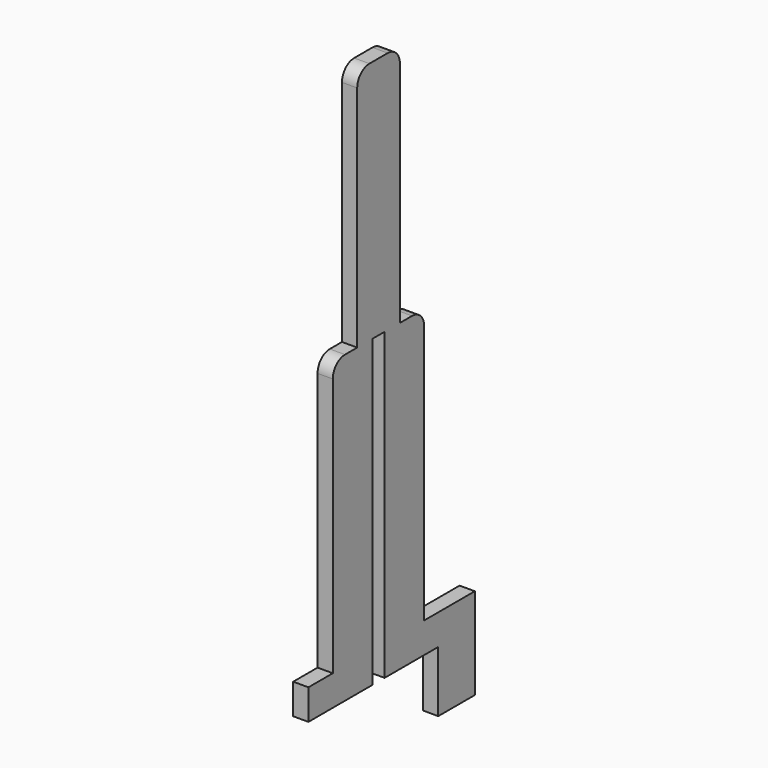
from build123d import *

# Parameters (mm, degrees)
F1_DEPTH = 3.175


# Not quite as in the source:
# - ends of sketch curves that miss each other by under 0.0002 mm in the source are joined


with BuildPart() as f1:
    # F0 (on Right) → F1 (new body, symmetric)
    with BuildSketch(Plane.YZ):
        with BuildLine():
            Line((3.175, -63.5), (23.8125, -63.5))
            Line((23.8125, -63.5), (23.8125, -50.8))
            Line((23.8125, -50.8), (23.8125, 57.15))
            ThreePointArc((23.8125, 57.15), (21.9533763667, 61.6393796296), (17.4646167058, 63.4999996472))
            Line((17.4646167058, 63.4999996472), (17.4625, 63.5))
            Line((17.4625, 63.5), (11.1139111112, 63.5))
            Line((11.1139111112, 63.5), (11.124494366, 158.7492930333))
            ThreePointArc((11.124494366, 158.7492930333), (9.2648719104, 163.2398771909), (4.7744944052, 165.0999985889))
            Line((4.7744944052, 165.0999985889), (-4.7498, 165.0999985889))
            ThreePointArc((-4.7498, 165.0999985889), (-9.2399280605, 163.2401266494), (-11.0998, 158.7499985889))
            Line((-11.0998, 158.7499985889), (-11.0998, 63.5))
            Line((-11.0998, 63.5), (-17.4498, 63.5))
            Line((-17.4498, 63.5), (-17.4625, 63.5))
            ThreePointArc((-17.4625, 63.5), (-21.9526280605, 61.6401280605), (-23.8125, 57.15))
            Line((-23.8125, 57.15), (-23.8125, -50.818807292))
            Line((-23.8125, -50.818807292), (-23.8125, -63.5))
            Line((-23.8125, -63.5), (-3.175, -63.5))
            Line((-3.175, -63.5), (-3.175, 63.5))
            Line((-3.175, 63.5), (3.175, 63.5))
            Line((3.175, 63.5), (3.175, -63.5))
        make_face()
        Polygon((23.8125, -50.8), (23.8125, -63.5), (31.115, -63.5), (31.115, -88.9), (50.165, -88.9), (50.165, -50.8), align=None)
        Polygon((-36.5125, -63.518807292), (-23.8125, -63.5), (-23.8125, -50.818807292), (-36.5125, -50.818807292), align=None)
    extrude(amount=F1_DEPTH, both=True)


solid = f1.part
